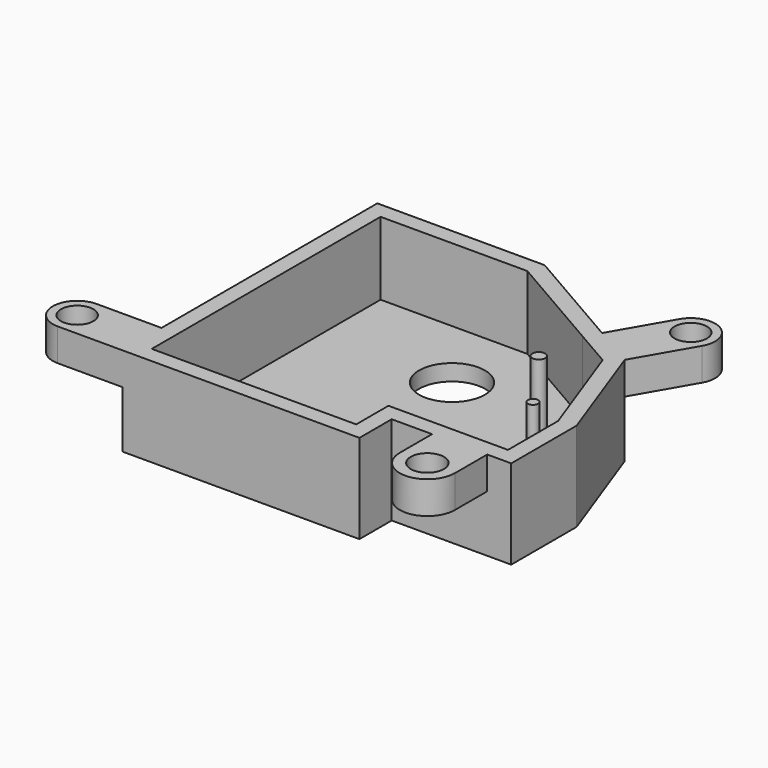
from build123d import *

# Parameters (mm, degrees)
F1_DEPTH = 17.4625
F2_T     = -3.175
F0_R     = 3.175
F0_R_2   = 3.25
F3_DEPTH = 6.35
F4_R     = 1
F4_R_2   = 1.25
F5_DEPTH = 14.2875
F4_R_3   = 6.45
F6_DEPTH = 3.176


# Not quite as in the source:
# - a feature names something its author has since deleted; it is built from what else it names


with BuildPart() as f1:
    # F0 (on Top) → F1 (new body)
    with BuildSketch(Plane.XY):
        Polygon((-32.7674517391, -39.2625403754), (13.6125482609, -39.2625403754), (13.6125482609, -31.3625403754), (21.5125482609, -31.3625403754), (32.3125482609, -31.3625403754), (37.0125482609, -31.3625403754), (37.0125482609, -15.3529706535), (29.1460849644, 6.2599596246), (20.8971929933, 11.0224596246), (0, 23.0874596246), (-32.7674517391, 23.0874596246), (-32.7674517391, -29.7375403754), align=None)
    extrude(amount=-F1_DEPTH)

    # F2
    f2_openings = [f1.faces().sort_by_distance(p)[0] for p in [
        (-2.028392, -9.399027, 0),
    ]]
    offset(amount=F2_T, openings=f2_openings, kind=Kind.INTERSECTION)

    # F0 (on Top) → F3 (join)
    with BuildSketch(Plane.XY):
        with BuildLine():
            Line((-45.4674517391, -39.2625403754), (-32.7674517391, -39.2625403754))
            Line((-32.7674517391, -39.2625403754), (-32.7674517391, -29.7375403754))
            Line((-32.7674517391, -29.7375403754), (-45.4674517391, -29.7375403754))
            ThreePointArc((-45.4674517391, -29.7375403754), (-50.2299517391, -34.5000403754), (-45.4674517391, -39.2625403754))
        make_face()
        with Locations((-45.4674517391, -34.5000403754)):
            Circle(F0_R, mode=Mode.SUBTRACT)
        with BuildLine():
            Line((27.2471929933, 22.0209822527), (20.8971929933, 11.0224596246))
            Line((20.8971929933, 11.0224596246), (29.1460849644, 6.2599596246))
            Line((29.1460849644, 6.2599596246), (35.4960849644, 17.2584822527))
            ThreePointArc((35.4960849644, 17.2584822527), (33.7528889788, 23.7641782382), (27.2471929933, 22.0209822527))
        make_face()
        with Locations((31.3716389788, 19.6397322527)):
            Circle(F0_R, mode=Mode.SUBTRACT)
        with BuildLine():
            Line((32.3125482609, -31.3625403754), (21.5125482609, -31.3625403754))
            Line((21.5125482609, -31.3625403754), (21.5125482609, -39.2625403754))
            ThreePointArc((21.5125482609, -39.2625403754), (26.9125482609, -44.6625403754), (32.3125482609, -39.2625403754))
            Line((32.3125482609, -39.2625403754), (32.3125482609, -31.3625403754))
        make_face()
        with Locations((26.9125482609, -39.2625403754)):
            Circle(F0_R_2, mode=Mode.SUBTRACT)
    extrude(amount=-F3_DEPTH)

    # F4 (on face) → F5 (join, through all)
    with BuildSketch(Plane.XY.offset(-14.2875)):
        with Locations((26.905224515, -13.3725403754)):
            Circle(F4_R)
        with Locations((18.055224515, -0.9225403754)):
            Circle(F4_R_2)
    extrude(amount=F5_DEPTH)

    # F4 (on face) → F6 (cut, through all)
    with BuildSketch(Plane.XY.offset(-14.2875)):
        with Locations((-3.9174517391, 5.3074596246)):
            Circle(F4_R_3)
    extrude(amount=-F6_DEPTH, mode=Mode.SUBTRACT)


solid = f1.part
